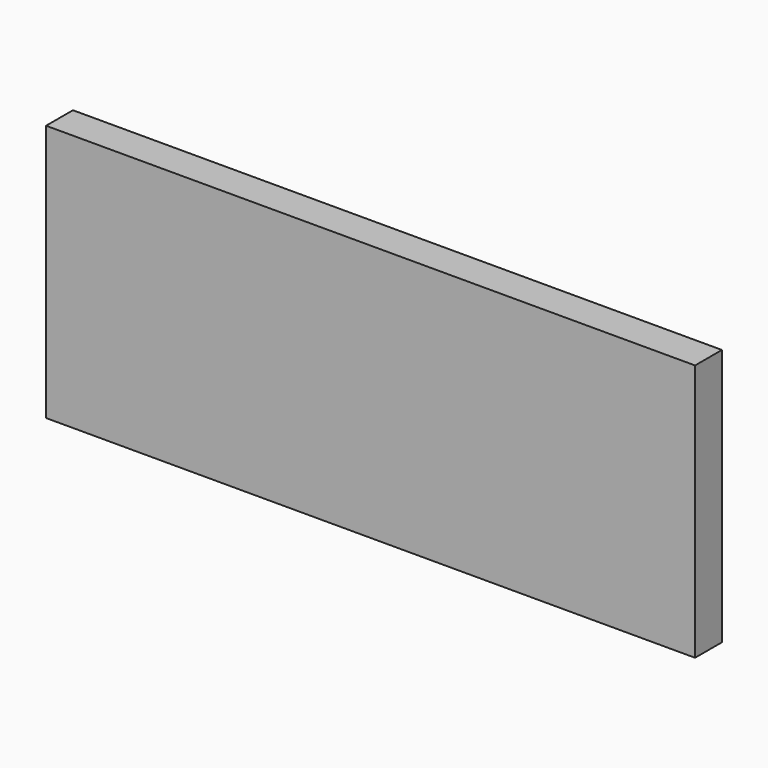
from build123d import *

# Parameters (mm, degrees)
F0_W     = 368.3
F0_H     = 146.05
F1_DEPTH = 19.05


# Not quite as in the source:
# - a length typed as a fraction of an inch, garbled in the dataset ("3 / 203.2 mm" for 3/8 in), is restored


with BuildPart() as f1:
    # F0 (on Front) → F1 (new body)
    with BuildSketch(Plane.XZ):
        with Locations((0.4225032568, -28.059548269)):
            Rectangle(F0_W, F0_H)
    extrude(amount=F1_DEPTH)


solid = f1.part
